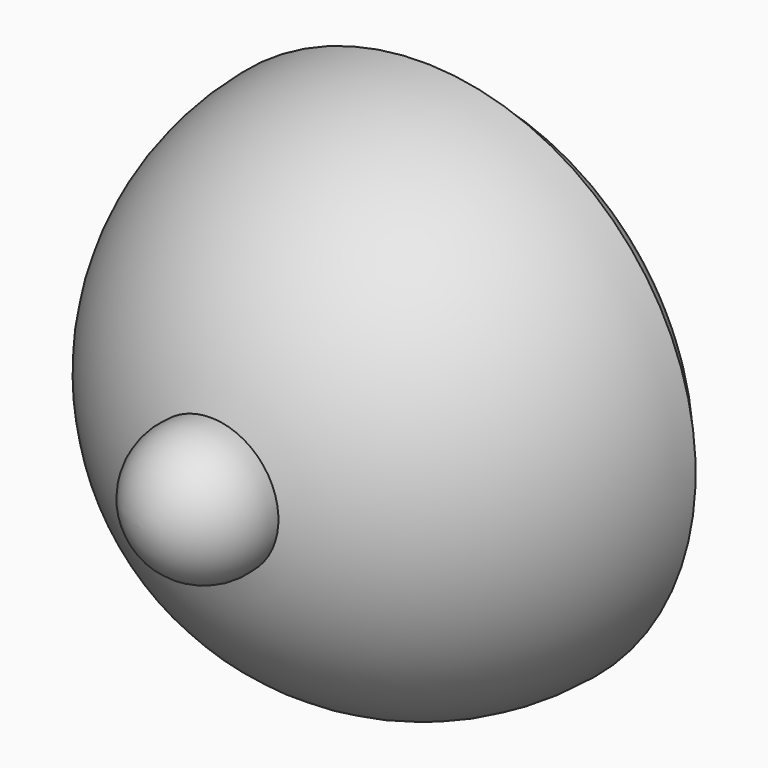
from build123d import *

# Parameters (mm, degrees)
F2_R     = 19
F3_DEPTH = 3
F4_R     = 2.99999


# Not quite as in the source:
# - a fillet or chamfer is up to 0.001 mm smaller than in the source, because OpenCascade refuses the exact size


with BuildPart() as f1:
    # F0 (on Top) → F1 (revolve)
    with BuildSketch(Plane.XY):
        with BuildLine():
            Line((0, 0), (-20, 0))
            ThreePointArc((-20, 0), (-15.7989821534, -12.2634482474), (-4.9607837082, -19.375))
            ThreePointArc((-4.9607837082, -19.375), (-3.75, -23.3071891388), (0, -25))
            Line((0, -25), (0, -20))
            Line((0, -20), (0, 0))
        make_face()
    revolve(axis=Axis((0, -10, 0), (0, -1, 0)))

    # F2 (on Front) → F3 (join)
    with BuildSketch(Plane.XZ):
        Circle(F2_R)
    extrude(amount=-F3_DEPTH)

    # F4 (radius 3 in the source; OpenCascade refuses exactly that, so slightly less here)
    f4_edges = [f1.edges().sort_by_distance(p)[0] for p in [
        (-19, 3, 0),
    ]]
    fillet(f4_edges, radius=F4_R)


solid = f1.part
